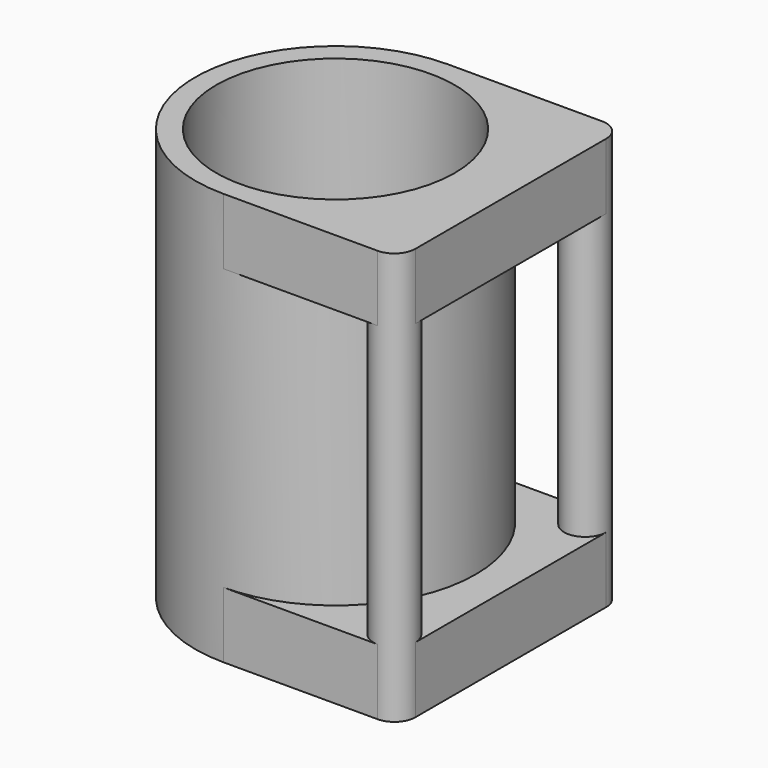
from build123d import *
from build123d import SkipClean  # not in build123d's __all__

# Parameters (mm, degrees)
F0_R        = 12.7
F0_R_2      = 10.795
F2_DEPTH    = 12.7
F2_FACE_R   = 1.905
F2_FACE_R_2 = 12.7
F2_FACE_R_3 = 10.795
F3_DEPTH    = 5.969


with BuildPart() as f2:
    # F0 (on Top) + F1 (on Top) → F2 (new body)
    with BuildSketch(Plane.XY):
        Circle(F0_R)
        Circle(F0_R_2, mode=Mode.SUBTRACT)
    with BuildSketch(Plane.XY):
        with BuildLine():
            ThreePointArc((15.8726907182, 10.795), (15.3147291364, 12.1420384182), (13.9676907182, 12.7))
            ThreePointArc((13.9676907182, 12.7), (12.6206523001, 9.4479615818), (15.8726907182, 10.795))
        make_face()
        with BuildLine():
            ThreePointArc((15.8726907182, -10.795), (12.6206523001, -9.4479615818), (13.9676907182, -12.7))
            ThreePointArc((13.9676907182, -12.7), (15.3147291364, -12.1420384182), (15.8726907182, -10.795))
        make_face()
    extrude(amount=F2_DEPTH)

    # F0 (on Top) + F1 (on Top) + F2_face (on face) → F3 (join)
    with BuildSketch(Plane.XY):
        Circle(F0_R)
        Circle(F0_R_2, mode=Mode.SUBTRACT)
    with BuildSketch(Plane.XY):
        with BuildLine():
            ThreePointArc((0, 12.7), (12.7, 0), (0, -12.7))
            Line((0, -12.7), (13.9676907182, -12.7))
            ThreePointArc((13.9676907182, -12.7), (12.6206523001, -9.4479615818), (15.8726907182, -10.795))
            Line((15.8726907182, -10.795), (15.8726907182, 10.795))
            ThreePointArc((15.8726907182, 10.795), (12.6206523001, 9.4479615818), (13.9676907182, 12.7))
            Line((13.9676907182, 12.7), (0, 12.7))
        make_face()
        with BuildLine():
            ThreePointArc((15.8726907182, -10.795), (12.6206523001, -9.4479615818), (13.9676907182, -12.7))
            ThreePointArc((13.9676907182, -12.7), (15.3147291364, -12.1420384182), (15.8726907182, -10.795))
        make_face()
        with BuildLine():
            ThreePointArc((15.8726907182, 10.795), (15.3147291364, 12.1420384182), (13.9676907182, 12.7))
            ThreePointArc((13.9676907182, 12.7), (12.6206523001, 9.4479615818), (15.8726907182, 10.795))
        make_face()
    with BuildSketch(Plane(origin=(13.9676907182, 10.795, 0), x_dir=(1, 0, 0), z_dir=(0, 0, -1))):
        Circle(F2_FACE_R)
        with Locations((-13.9676907182, 10.795)):
            Circle(F2_FACE_R_2)
        with Locations((-13.9676907182, 10.795)):
            Circle(F2_FACE_R_3, mode=Mode.SUBTRACT)
        with Locations((0, 21.59)):
            Circle(F2_FACE_R)
    with SkipClean():  # cleaning this boolean's faces spoils the solid; the shape is the same uncleaned
        extrude(amount=-F3_DEPTH, dir=(0, 0, 1))

    # F5: F2 across plane


with BuildPart() as f2_1:
    add(f2.part, clean=False)
    add(f2.part.mirror(Plane.XY.offset(12.7)), clean=False)


solid = f2_1.part
